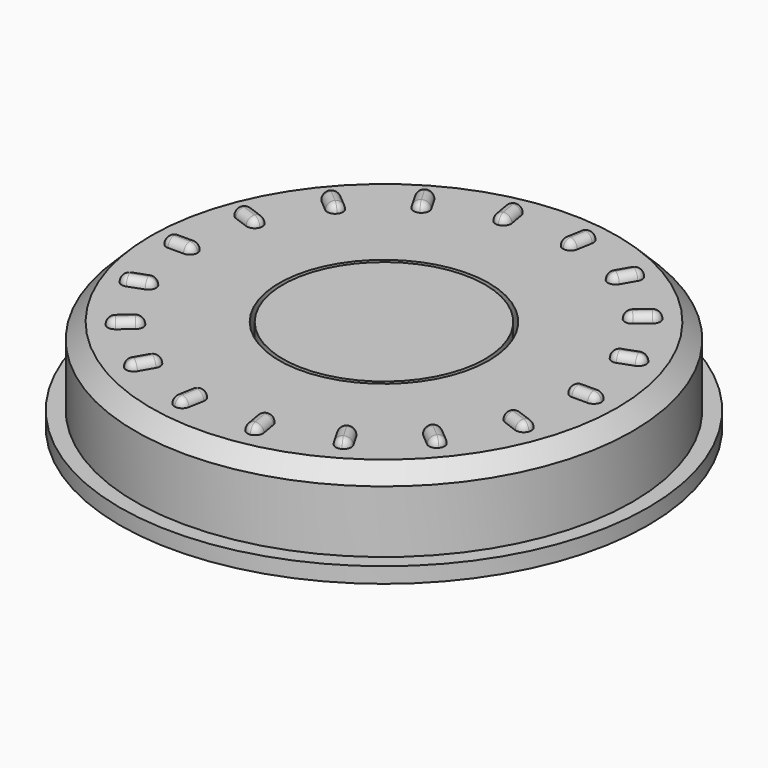
from build123d import *

# Parameters (mm, degrees)
F0_R      = 17
F1_DEPTH  = 1
F2_R      = 16
F3_DEPTH  = 5
F4_SIZE   = 1
F5_R      = 6.75
F6_DEPTH  = 3
F7_R      = 6.5
F8_DEPTH  = 2.5
F9_W      = 2
F9_H      = 1
F10_DEPTH = 0.5
F11_R     = 0.49999
F12_R     = 0.49999
F13_R     = 0.49999
F14_R     = 0.49999
F15_R     = 0.49999
F16_R     = 0.49999
F17_R     = 0.49999
F18_R     = 0.49999
F19_R     = 0.49999
F20_R     = 0.49999
F21_R     = 0.49999
F22_R     = 0.49999
F23_R     = 0.49999
F24_R     = 0.49999
F25_R     = 0.49999
F26_R     = 0.49999
F27_R     = 0.49999
F28_R     = 0.49999
F29_R     = 9.26
F30_DEPTH = 1.25
F31_R     = 0.75
F32_DEPTH = 1.5
F33_SIZE  = 0.2
F34_W     = 1.2
F34_H     = 0.2
F34_W_2   = 0.2
F34_H_2   = 1.2
F35_DEPTH = 3.5
F36_R     = 0.59999


# Not quite as in the source:
# - a fillet or chamfer is up to 0.001 mm smaller than in the source, because OpenCascade refuses the exact size


with BuildPart() as f1:
    # F0 (on Top) → F1 (new body)
    with BuildSketch(Plane.XY):
        Circle(F0_R)
    extrude(amount=F1_DEPTH)

    # F2 (on face) → F3 (join)
    with BuildSketch(Plane.XY.offset(1)):
        Circle(F2_R)
    extrude(amount=F3_DEPTH)

    # F4
    f4_edges = [f1.edges().sort_by_distance(p)[0] for p in [
        (-16, 0, 6),
    ]]
    chamfer(f4_edges, length=F4_SIZE)

    # F5 (on face) → F6 (cut)
    with BuildSketch(Plane.XY.offset(6)):
        Circle(F5_R)
    extrude(amount=-F6_DEPTH, mode=Mode.SUBTRACT)

    # F9 (on face) → F10 (join)
    with BuildSketch(Plane.XY.offset(6)):
        with Locations((13, 0)):
            Rectangle(F9_W, F9_H)
        Polygon((12.9846866193, 5.258128317), (11.1053013778, 4.5740880303), (11.4473215211, 3.6343954095), (13.3267067627, 4.3184356962), align=None)
        Polygon((10.4032283988, 9.3820487572), (8.8711395126, 8.0964735378), (9.5139271223, 7.3304290947), (11.0460160085, 8.6160043141), align=None)
        Polygon((6.5669872981, 12.374355653), (5.5669872981, 10.6423048454), (6.4330127019, 10.1423048454), (7.4330127019, 11.874355653), align=None)
        Polygon((1.9386706108, 13.874132631), (1.5913742555, 11.904517125), (2.5761820085, 11.7308689473), (2.9234783638, 13.7004844533), align=None)
        Polygon((-2.9234783638, 13.7004844533), (-2.5761820085, 11.7308689473), (-1.5913742555, 11.904517125), (-1.9386706108, 13.874132631), align=None)
        Polygon((-7.4330127019, 11.874355653), (-6.4330127019, 10.1423048454), (-5.5669872981, 10.6423048454), (-6.5669872981, 12.374355653), align=None)
        Polygon((-11.0460160085, 8.6160043141), (-9.5139271223, 7.3304290947), (-8.8711395126, 8.0964735378), (-10.4032283988, 9.3820487572), align=None)
        Polygon((-13.3267067627, 4.3184356962), (-11.4473215211, 3.6343954095), (-11.1053013778, 4.5740880303), (-12.9846866193, 5.258128317), align=None)
        with Locations((-13, 0)):
            Rectangle(F9_W, F9_H)
        Polygon((-12.9846866193, -5.258128317), (-11.1053013778, -4.5740880303), (-11.4473215211, -3.6343954095), (-13.3267067627, -4.3184356962), align=None)
        Polygon((-10.4032283988, -9.3820487572), (-8.8711395126, -8.0964735378), (-9.5139271223, -7.3304290947), (-11.0460160085, -8.6160043141), align=None)
        Polygon((-6.5669872981, -12.374355653), (-5.5669872981, -10.6423048454), (-6.4330127019, -10.1423048454), (-7.4330127019, -11.874355653), align=None)
        Polygon((-1.9386706108, -13.874132631), (-1.5913742555, -11.904517125), (-2.5761820085, -11.7308689473), (-2.9234783638, -13.7004844533), align=None)
        Polygon((2.9234783638, -13.7004844533), (2.5761820085, -11.7308689473), (1.5913742555, -11.904517125), (1.9386706108, -13.874132631), align=None)
        Polygon((7.4330127019, -11.874355653), (6.4330127019, -10.1423048454), (5.5669872981, -10.6423048454), (6.5669872981, -12.374355653), align=None)
        Polygon((11.0460160085, -8.6160043141), (9.5139271223, -7.3304290947), (8.8711395126, -8.0964735378), (10.4032283988, -9.3820487572), align=None)
        Polygon((13.3267067627, -4.3184356962), (11.4473215211, -3.6343954095), (11.1053013778, -4.5740880303), (12.9846866193, -5.258128317), align=None)
    extrude(amount=F10_DEPTH)

    # F11 (radius 0.5 in the source; OpenCascade refuses exactly that, so slightly less here)
    f11_edges = [f1.edges().sort_by_distance(p)[0] for p in [
        (14, -0.5, 6.25),
        (14, 0.5, 6.25),
        (12, -0.5, 6.25),
        (12, 0.5, 6.25),
        (13, 0.5, 6.5),
        (13, -0.5, 6.5),
        (12, 0, 6.5),
        (14, 0, 6.5),
    ]]
    fillet(f11_edges, radius=F11_R)

    # F12 (radius 0.5 in the source; OpenCascade refuses exactly that, so slightly less here)
    f12_edges = [f1.edges().sort_by_distance(p)[0] for p in [
        (12.984687, 5.258128, 6.25),
        (13.326707, 4.318436, 6.25),
        (11.105301, 4.574088, 6.25),
        (11.447322, 3.634395, 6.25),
        (12.387014, 3.976416, 6.5),
        (12.044994, 4.916108, 6.5),
        (11.276311, 4.104242, 6.5),
        (13.155697, 4.788282, 6.5),
    ]]
    fillet(f12_edges, radius=F12_R)

    # F13 (radius 0.5 in the source; OpenCascade refuses exactly that, so slightly less here)
    f13_edges = [f1.edges().sort_by_distance(p)[0] for p in [
        (12.984687, -5.258128, 6.25),
        (13.326707, -4.318436, 6.25),
        (11.105301, -4.574088, 6.25),
        (11.447322, -3.634395, 6.25),
        (12.387014, -3.976416, 6.5),
        (12.044994, -4.916108, 6.5),
        (13.155697, -4.788282, 6.5),
        (11.276311, -4.104242, 6.5),
    ]]
    fillet(f13_edges, radius=F13_R)

    # F14 (radius 0.5 in the source; OpenCascade refuses exactly that, so slightly less here)
    f14_edges = [f1.edges().sort_by_distance(p)[0] for p in [
        (10.403228, -9.382049, 6.25),
        (11.046016, -8.616004, 6.25),
        (8.87114, -8.096474, 6.25),
        (9.513927, -7.330429, 6.25),
        (10.279972, -7.973217, 6.5),
        (9.637184, -8.739261, 6.5),
        (10.724622, -8.999027, 6.5),
        (9.192533, -7.713451, 6.5),
    ]]
    fillet(f14_edges, radius=F14_R)

    # F15 (radius 0.5 in the source; OpenCascade refuses exactly that, so slightly less here)
    f15_edges = [f1.edges().sort_by_distance(p)[0] for p in [
        (7.433013, -11.874356, 6.25),
        (6.433013, -10.142305, 6.25),
        (6.566987, -12.374356, 6.25),
        (5.566987, -10.642305, 6.25),
        (6.066987, -11.50833, 6.5),
        (6.933013, -11.00833, 6.5),
        (7, -12.124356, 6.5),
        (6, -10.392305, 6.5),
    ]]
    fillet(f15_edges, radius=F15_R)

    # F16 (radius 0.5 in the source; OpenCascade refuses exactly that, so slightly less here)
    f16_edges = [f1.edges().sort_by_distance(p)[0] for p in [
        (1.591374, -11.904517, 6.25),
        (1.938671, -13.874133, 6.25),
        (2.923478, -13.700484, 6.25),
        (2.576182, -11.730869, 6.25),
        (1.765022, -12.889325, 6.5),
        (2.74983, -12.715677, 6.5),
        (2.431074, -13.787309, 6.5),
        (2.083778, -11.817693, 6.5),
    ]]
    fillet(f16_edges, radius=F16_R)

    # F17 (radius 0.5 in the source; OpenCascade refuses exactly that, so slightly less here)
    f17_edges = [f1.edges().sort_by_distance(p)[0] for p in [
        (-2.923478, -13.700484, 6.25),
        (-1.938671, -13.874133, 6.25),
        (-2.576182, -11.730869, 6.25),
        (-1.591374, -11.904517, 6.25),
        (-1.765022, -12.889325, 6.5),
        (-2.74983, -12.715677, 6.5),
        (-2.431074, -13.787309, 6.5),
        (-2.083778, -11.817693, 6.5),
    ]]
    fillet(f17_edges, radius=F17_R)

    # F18 (radius 0.5 in the source; OpenCascade refuses exactly that, so slightly less here)
    f18_edges = [f1.edges().sort_by_distance(p)[0] for p in [
        (-7.433013, -11.874356, 6.25),
        (-6.566987, -12.374356, 6.25),
        (-6.433013, -10.142305, 6.25),
        (-5.566987, -10.642305, 6.25),
        (-6.933013, -11.00833, 6.5),
        (-6.066987, -11.50833, 6.5),
        (-7, -12.124356, 6.5),
        (-6, -10.392305, 6.5),
    ]]
    fillet(f18_edges, radius=F18_R)

    # F19 (radius 0.5 in the source; OpenCascade refuses exactly that, so slightly less here)
    f19_edges = [f1.edges().sort_by_distance(p)[0] for p in [
        (-11.046016, -8.616004, 6.25),
        (-10.403228, -9.382049, 6.25),
        (-9.513927, -7.330429, 6.25),
        (-8.87114, -8.096474, 6.25),
        (-9.637184, -8.739261, 6.5),
        (-10.279972, -7.973217, 6.5),
        (-9.192533, -7.713451, 6.5),
        (-10.724622, -8.999027, 6.5),
    ]]
    fillet(f19_edges, radius=F19_R)

    # F20 (radius 0.5 in the source; OpenCascade refuses exactly that, so slightly less here)
    f20_edges = [f1.edges().sort_by_distance(p)[0] for p in [
        (-13.326707, -4.318436, 6.25),
        (-12.984687, -5.258128, 6.25),
        (-11.447322, -3.634395, 6.25),
        (-11.105301, -4.574088, 6.25),
        (-12.044994, -4.916108, 6.5),
        (-12.387014, -3.976416, 6.5),
        (-11.276311, -4.104242, 6.5),
        (-13.155697, -4.788282, 6.5),
    ]]
    fillet(f20_edges, radius=F20_R)

    # F21 (radius 0.5 in the source; OpenCascade refuses exactly that, so slightly less here)
    f21_edges = [f1.edges().sort_by_distance(p)[0] for p in [
        (-14, 0.5, 6.25),
        (-14, -0.5, 6.25),
        (-12, 0.5, 6.25),
        (-12, -0.5, 6.25),
        (-13, -0.5, 6.5),
        (-13, 0.5, 6.5),
        (-12, 0, 6.5),
        (-14, 0, 6.5),
    ]]
    fillet(f21_edges, radius=F21_R)

    # F22 (radius 0.5 in the source; OpenCascade refuses exactly that, so slightly less here)
    f22_edges = [f1.edges().sort_by_distance(p)[0] for p in [
        (-13.326707, 4.318436, 6.25),
        (-12.984687, 5.258128, 6.25),
        (-11.447322, 3.634395, 6.25),
        (-11.105301, 4.574088, 6.25),
        (-12.387014, 3.976416, 6.5),
        (-12.044994, 4.916108, 6.5),
        (-11.276311, 4.104242, 6.5),
        (-13.155697, 4.788282, 6.5),
    ]]
    fillet(f22_edges, radius=F22_R)

    # F23 (radius 0.5 in the source; OpenCascade refuses exactly that, so slightly less here)
    f23_edges = [f1.edges().sort_by_distance(p)[0] for p in [
        (-11.046016, 8.616004, 6.25),
        (-10.403228, 9.382049, 6.25),
        (-9.513927, 7.330429, 6.25),
        (-8.87114, 8.096474, 6.25),
        (-10.279972, 7.973217, 6.5),
        (-9.637184, 8.739261, 6.5),
        (-9.192533, 7.713451, 6.5),
        (-10.724622, 8.999027, 6.5),
    ]]
    fillet(f23_edges, radius=F23_R)

    # F24 (radius 0.5 in the source; OpenCascade refuses exactly that, so slightly less here)
    f24_edges = [f1.edges().sort_by_distance(p)[0] for p in [
        (-7.433013, 11.874356, 6.25),
        (-6.433013, 10.142305, 6.25),
        (-6.566987, 12.374356, 6.25),
        (-5.566987, 10.642305, 6.25),
        (-6.066987, 11.50833, 6.5),
        (-6.933013, 11.00833, 6.5),
        (-6, 10.392305, 6.5),
        (-7, 12.124356, 6.5),
    ]]
    fillet(f24_edges, radius=F24_R)

    # F25 (radius 0.5 in the source; OpenCascade refuses exactly that, so slightly less here)
    f25_edges = [f1.edges().sort_by_distance(p)[0] for p in [
        (-2.923478, 13.700484, 6.25),
        (-2.576182, 11.730869, 6.25),
        (-1.591374, 11.904517, 6.25),
        (-1.938671, 13.874133, 6.25),
        (-1.765022, 12.889325, 6.5),
        (-2.74983, 12.715677, 6.5),
        (-2.083778, 11.817693, 6.5),
        (-2.431074, 13.787309, 6.5),
    ]]
    fillet(f25_edges, radius=F25_R)

    # F26 (radius 0.5 in the source; OpenCascade refuses exactly that, so slightly less here)
    f26_edges = [f1.edges().sort_by_distance(p)[0] for p in [
        (1.938671, 13.874133, 6.25),
        (1.591374, 11.904517, 6.25),
        (2.576182, 11.730869, 6.25),
        (2.923478, 13.700484, 6.25),
        (2.74983, 12.715677, 6.5),
        (1.765022, 12.889325, 6.5),
        (2.083778, 11.817693, 6.5),
        (2.431074, 13.787309, 6.5),
    ]]
    fillet(f26_edges, radius=F26_R)

    # F27 (radius 0.5 in the source; OpenCascade refuses exactly that, so slightly less here)
    f27_edges = [f1.edges().sort_by_distance(p)[0] for p in [
        (5.566987, 10.642305, 6.25),
        (6.433013, 10.142305, 6.25),
        (6.566987, 12.374356, 6.25),
        (7.433013, 11.874356, 6.25),
        (6.933013, 11.00833, 6.5),
        (7, 12.124356, 6.5),
        (6.066987, 11.50833, 6.5),
        (6, 10.392305, 6.5),
    ]]
    fillet(f27_edges, radius=F27_R)

    # F28 (radius 0.5 in the source; OpenCascade refuses exactly that, so slightly less here)
    f28_edges = [f1.edges().sort_by_distance(p)[0] for p in [
        (10.403228, 9.382049, 6.25),
        (11.046016, 8.616004, 6.25),
        (9.513927, 7.330429, 6.25),
        (8.87114, 8.096474, 6.25),
        (9.637184, 8.739261, 6.5),
        (10.279972, 7.973217, 6.5),
        (9.192533, 7.713451, 6.5),
        (10.724622, 8.999027, 6.5),
    ]]
    fillet(f28_edges, radius=F28_R)

    # F29 (on face) → F30 (join)
    with BuildSketch(Plane(origin=(0, 0, 0), x_dir=(1, 0, 0), z_dir=(0, 0, -1))):
        Circle(F29_R)
    extrude(amount=F30_DEPTH)

    # F31 (on face) → F32 (join)
    with BuildSketch(Plane(origin=(0, 0, -1.25), x_dir=(1, 0, 0), z_dir=(0, 0, -1))):
        with Locations((-4.5, 0)):
            Circle(F31_R)
        with Locations((4.5, 0)):
            Circle(F31_R)
    extrude(amount=F32_DEPTH)

    # F33
    f33_edges = [f1.edges().sort_by_distance(p)[0] for p in [
        (-5.25, 0, -2.75),
        (3.75, 0, -2.75),
    ]]
    chamfer(f33_edges, length=F33_SIZE)

    # F34 (on face) → F35 (join)
    with BuildSketch(Plane(origin=(0, 0, -1.25), x_dir=(1, 0, 0), z_dir=(0, 0, -1))):
        with Locations((0, -9.26)):
            Rectangle(F34_W, F34_H)
        with Locations((0, 1.57)):
            Rectangle(F34_W, F34_H)
        with Locations((-9.26, 0)):
            Rectangle(F34_W_2, F34_H_2)
        with Locations((9.26, 0)):
            Rectangle(F34_W_2, F34_H_2)
    extrude(amount=F35_DEPTH)

    # F36 (radius 0.6 in the source; OpenCascade refuses exactly that, so slightly less here)
    f36_edges = [f1.edges().sort_by_distance(p)[0] for p in [
        (0.6, -1.57, -4.75),
        (-0.6, -1.57, -4.75),
        (-0.6, 9.26, -4.75),
        (0.6, 9.26, -4.75),
        (9.26, -0.6, -4.75),
        (9.26, 0.6, -4.75),
        (-9.26, 0.6, -4.75),
        (-9.26, -0.6, -4.75),
    ]]
    fillet(f36_edges, radius=F36_R)


with BuildPart() as f8:
    # F7 (on face) → F8 (new body)
    with BuildSketch(Plane.XY.offset(6)):
        Circle(F7_R)
    extrude(amount=-F8_DEPTH)


solid = Compound([f1.part, f8.part])
